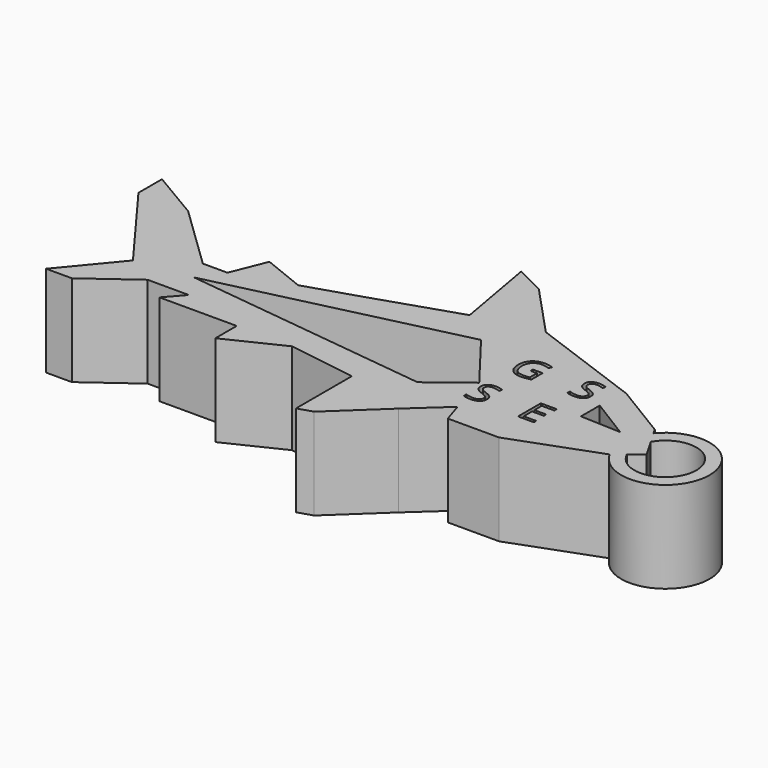
from build123d import *

# Parameters (mm, degrees)
F1_DEPTH     = 12.7
F2_R         = 6.1366625173
F2_R_2       = 4.3074098206
F3_DEPTH     = 12.7
F4_TEXT_SIZE = 5.5429622686
F5_DEPTH     = 5


# Not quite as in the source:
# - Text() gives the source's letters only with a copy of the font that has no kerning and outlines rounded to 1/6400 em; it was checked with that copy


with BuildPart() as f1:
    # F0 (on Top) → F1 (new body)
    with BuildSketch(Plane.XY):
        Polygon((38.4212136269, 0), (22.5748755038, 5.8197807521), (15.6740508974, 13.2317766547), (11.5846730769, 15.276465565), (13.6293638498, 3.7750927731), (2.1279922221, 0), (-5.284007173, -2.3589723278), (-11.1624840647, 0), (-13.1099203575, -4.8529434238), (-16.5297929198, -4.8529434238), (-25.4753045738, 3.7750927731), (-32.3761254549, 7.8644696623), (-32.3761254549, 3.7750927731), (-22.9194443673, -9.0042091906), (-29.0535073727, -16.4162050933), (-25.4753045738, -16.4162050933), (-18.8300665468, -11.5600703284), (-13.1099203575, -11.5600703284), (-15.2518618852, -13.9881377108), (-9.8845539615, -13.9881377108), (-4.5172460377, -13.9881377108), (-4.5172460377, -17.6941342652), (3.1503352802, -13.9881377108), (12.6070166007, -15.3938606381), (12.6070166007, -25.1061301678), (14.6323512997, -24.4615391129), (21.2969463319, -18.2053074241), (26.0613807593, -13.8641195372), (26.9557219243, -16.6741805525), (34.0762473643, -16.6741805525), (45.8332039416, -12.330035679), (49.0831501688, -9.8324515542), (46.0887923837, -4.6596103348), align=None)
        Polygon((-15.2518618852, -7.9818656668), (18.2299111038, 0), (24.3639759719, -7.9818656668), (19.0509699686, -12.0649115147), align=None, mode=Mode.SUBTRACT)
        Polygon((37.910040468, -7.2460309445), (37.910040468, -3.9909328334), (43.5329340398, -7.4720992707), align=None, mode=Mode.SUBTRACT)
    extrude(amount=F1_DEPTH)

    # F2 (on Top) → F3 (join)
    with BuildSketch(Plane.XY):
        with Locations((51.2942895293, -9.3193463981)):
            Circle(F2_R)
        with Locations((51.2942895293, -9.3193463981)):
            Circle(F2_R_2, mode=Mode.SUBTRACT)
    extrude(amount=F3_DEPTH)

    # F4 (on face) → F5 (cut)
    with BuildSketch(Plane.XY.offset(12.7)):
        with Locations((24.684112519, -3.9909328334)):
            Text('G   S', F4_TEXT_SIZE, font='Open Sans', text_align=(TextAlign.LEFT, TextAlign.BOTTOM))
        with Locations((24.684112519, -11.5293615187)):
            Text('S   E', F4_TEXT_SIZE, font='Open Sans', text_align=(TextAlign.LEFT, TextAlign.BOTTOM))
    extrude(amount=-F5_DEPTH, mode=Mode.SUBTRACT)


solid = f1.part
